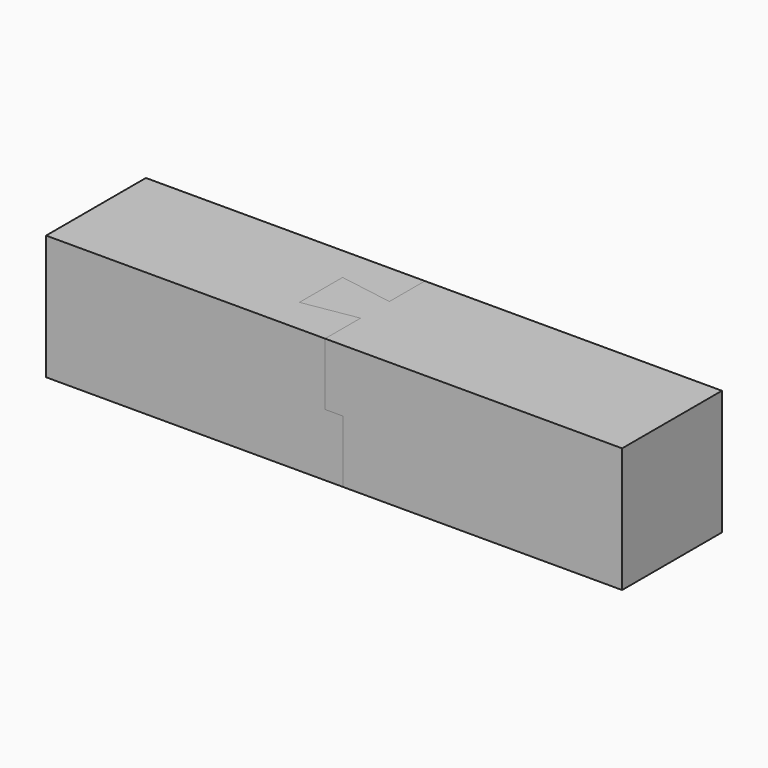
from build123d import *

# Parameters (mm, degrees)
F0_W          = 250
F0_H          = 105
F1_DEPTH      = 52.5
F2_W          = 105
F2_H          = 52.5
F3_DEPTH      = 15.15
F5_DEPTH      = 52.5
F6_W          = 250
F6_H          = 105
F7_DEPTH      = 52.5
F7_DEPTH_BACK = 52.5


with BuildPart() as f1:
    # F0 (on Top) → F1 (new body, symmetric)
    with BuildSketch(Plane.XY):
        with Locations((125, 0)):
            Rectangle(F0_W, F0_H)
    extrude(amount=F1_DEPTH, both=True)

    # F2 (on face) → F3 (cut)
    with BuildSketch(Plane(origin=(0, 0, 0), x_dir=(0, -1, 0), z_dir=(-1, 0, 0))):
        with Locations((0, -26.25)):
            Rectangle(F2_W, F2_H)
    extrude(amount=-F3_DEPTH, mode=Mode.SUBTRACT)

    # F4 (on face) → F5 (join, through all)
    with BuildSketch(Plane.XY.offset(52.5)):
        Polygon((0, -15.15), (0, 15.15), (-45.45, 22.725), (-45.45, -22.725), align=None)
    extrude(amount=-F5_DEPTH)


with BuildPart() as f7:
    # F6 (on Top) → F7 (new body, two sides)
    with BuildSketch(Plane.XY) as f7_sk:
        with Locations((-109.85, 0)):
            Rectangle(F6_W, F6_H)
    extrude(amount=F7_DEPTH)
    extrude(f7_sk.sketch, amount=-F7_DEPTH_BACK)

    # F8: cut F1
    add(f1.part, mode=Mode.SUBTRACT)


solid = Compound([f1.part, f7.part])
